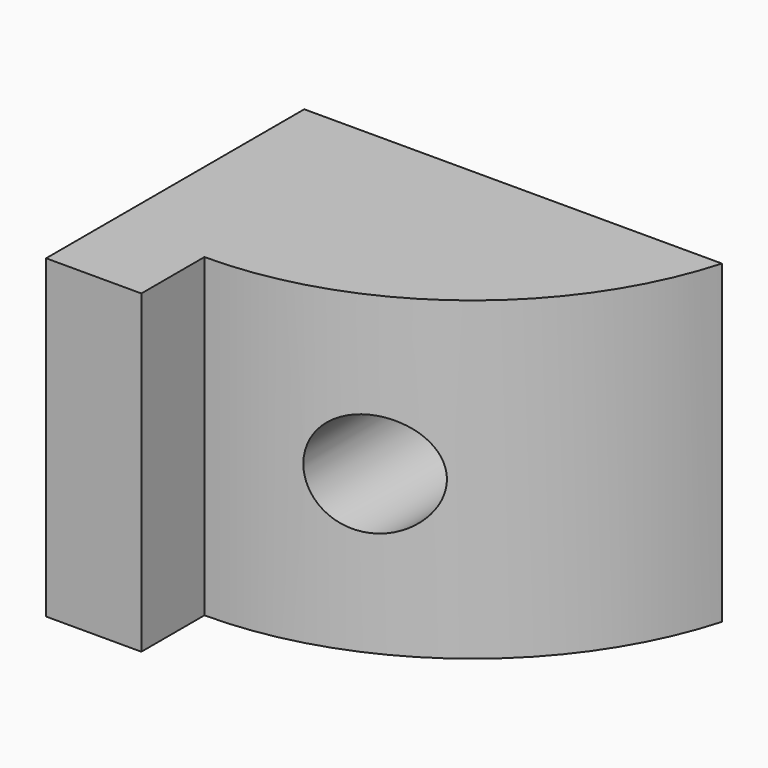
from build123d import *

# Parameters (mm, degrees)
F0_W        = 33.6334481835
F0_H        = 19.636919722
F1_DEPTH    = 25.4
F2_T1_DEPTH = 155.2122388964
F3_R        = 4.1932918126
F4_DEPTH    = 41.402
F5_DEPTH    = 6.35


# Not quite as in the source:
# - a fillet or chamfer that OpenCascade refuses, or shapes differently, is made with other operations: its cross-section is extruded or revolved along the edge and cut away or added


with BuildPart() as f1:
    # F0 (on Top) → F1 (new body)
    with BuildSketch(Plane.XY):
        with Locations((-16.8167240918, 9.818459861)):
            Rectangle(F0_W, F0_H)
    extrude(amount=F1_DEPTH)

    # F2: fillet of radius 26.9812507731 on 1 edges, made by hand

    # F2_s2 → F2_t1 (cut)
    with BuildSketch(Plane.XY.offset(-64.9061194482)):
        with BuildLine():
            ThreePointArc((-25.9624477793, 0), (-9.6862587992, 5.4621066087), (0, 19.636919722))
            Line((0, 19.636919722), (0, 0))
            Line((0, 0), (-25.9624477793, 0))
        make_face()
    extrude(amount=F2_T1_DEPTH, mode=Mode.SUBTRACT)

    # F3 (on face) → F4 (cut)
    with BuildSketch(Plane(origin=(0, 19.636919722, 0), x_dir=(-1, 0, 0), z_dir=(0, 1, 0))):
        with Locations((14.5834481835, 12.7)):
            Circle(F3_R)
    extrude(amount=-F4_DEPTH, mode=Mode.SUBTRACT)

    # F5 (add): a face of the model
    f5_faces = [f1.faces().sort_by_distance(p)[0] for p in [
        (-29.7979479814, 0, 12.7),
    ]]
    extrude(f5_faces, amount=F5_DEPTH)


solid = f1.part
